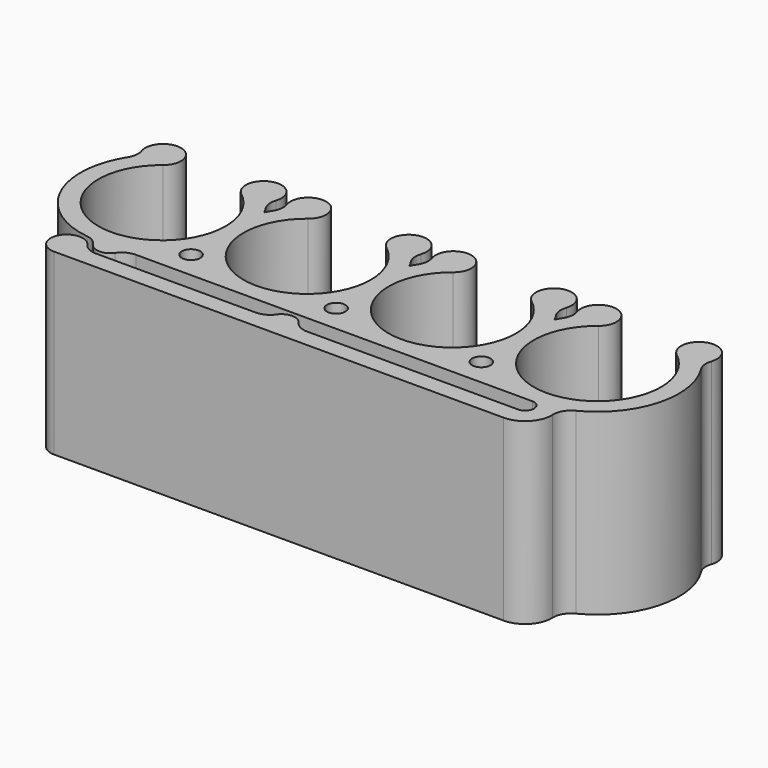
from build123d import *

# Parameters (mm, degrees)
F1_R     = 1.03125
F2_DEPTH = 10
F3_R     = 2


with BuildPart() as f2:
    # F1 (on Top) → F2 (new body, symmetric)
    with BuildSketch(Plane.XY):
        with BuildLine():
            ThreePointArc((-19.9828767123, 14.7352475904), (-17.9695529655, 12.2452360949), (-17.25, 9.125))
            ThreePointArc((-17.25, 9.125), (-27.4952360949, 2.7195529655), (-28.7671232877, 14.7352475904))
            ThreePointArc((-28.7671232877, 14.7352475904), (-29.8675330526, 18.3056622368), (-31.4302114786, 14.9120213402))
            ThreePointArc((-31.4302114786, 14.9120213402), (-32.6233996851, 5.2224972601), (-24.375, 0))
            Line((-24.375, 0), (-21.375, 0))
            Line((-21.375, 0), (24.375, 0))
            ThreePointArc((24.375, 0), (25.7175606637, 0.099305796), (27.0308996167, 0.3950617284))
            ThreePointArc((27.0308996167, 0.3950617284), (33.107808756, 6.4785540378), (31.4302114786, 14.9120213402))
            ThreePointArc((31.4302114786, 14.9120213402), (29.8675330526, 18.3056622368), (28.7671232877, 14.7352475904))
            ThreePointArc((28.7671232877, 14.7352475904), (30.7804470345, 12.2452360949), (31.5, 9.125))
            ThreePointArc((31.5, 9.125), (21.2547639051, 2.7195529655), (19.9828767123, 14.7352475904))
            ThreePointArc((19.9828767123, 14.7352475904), (18.8824669474, 18.3056622368), (17.3197885214, 14.9120213402))
            ThreePointArc((17.3197885214, 14.9120213402), (16.7410654482, 14.1238666974), (16.25, 13.2783119315))
            ThreePointArc((16.25, 13.2783119315), (15.7589345518, 14.1238666974), (15.1802114786, 14.9120213402))
            ThreePointArc((15.1802114786, 14.9120213402), (13.6175330526, 18.3056622368), (12.5171232877, 14.7352475904))
            ThreePointArc((12.5171232877, 14.7352475904), (14.5304470345, 12.2452360949), (15.25, 9.125))
            ThreePointArc((15.25, 9.125), (5.0047639051, 2.7195529655), (3.7328767123, 14.7352475904))
            ThreePointArc((3.7328767123, 14.7352475904), (2.6324669474, 18.3056622368), (1.0697885214, 14.9120213402))
            ThreePointArc((1.0697885214, 14.9120213402), (0.4910654482, 14.1238666974), (0, 13.2783119315))
            ThreePointArc((0, 13.2783119315), (-0.4910654482, 14.1238666974), (-1.0697885214, 14.9120213402))
            ThreePointArc((-1.0697885214, 14.9120213402), (-2.6324669474, 18.3056622368), (-3.7328767123, 14.7352475904))
            ThreePointArc((-3.7328767123, 14.7352475904), (-1.7195529655, 12.2452360949), (-1, 9.125))
            ThreePointArc((-1, 9.125), (-11.2452360949, 2.7195529655), (-12.5171232877, 14.7352475904))
            ThreePointArc((-12.5171232877, 14.7352475904), (-13.6175330526, 18.3056622368), (-15.1802114786, 14.9120213402))
            ThreePointArc((-15.1802114786, 14.9120213402), (-15.7589345518, 14.1238666974), (-16.25, 13.2783119315))
            ThreePointArc((-16.25, 13.2783119315), (-16.7410654482, 14.1238666974), (-17.3197885214, 14.9120213402))
            ThreePointArc((-17.3197885214, 14.9120213402), (-18.8824669474, 18.3056622368), (-19.9828767123, 14.7352475904))
        make_face()
        with Locations((-16.25, 3.03125)):
            Circle(F1_R, mode=Mode.SUBTRACT)
        with Locations((0, 3.03125)):
            Circle(F1_R, mode=Mode.SUBTRACT)
        with Locations((16.25, 3.03125)):
            Circle(F1_R, mode=Mode.SUBTRACT)
        with BuildLine():
            ThreePointArc((27.0308996167, 0.3950617284), (25.7175606637, 0.099305796), (24.375, 0))
            ThreePointArc((24.375, 0), (25.375, -1), (24.375, -2))
            Line((24.375, -2), (-0.6061253537, -2))
            Line((-0.6061253537, -2), (-3.6061253537, -2))
            Line((-3.6061253537, -2), (-24.1903478035, -2))
            ThreePointArc((-24.1903478035, -2), (-27.3314384085, -0.985167759), (-25.9871463178, -4))
            Line((-25.9871463178, -4), (24.375, -4))
            ThreePointArc((24.375, -4), (26.9426044463, -2.5515822271), (27.0308996167, 0.3950617284))
        make_face()
        with BuildLine():
            Line((-21.375, 0), (-24.375, 0))
            ThreePointArc((-24.375, 0), (-22.875, -1.5), (-21.375, 0))
        make_face()
        with BuildLine():
            Line((-3.6061253537, -2), (-0.6061253537, -2))
            ThreePointArc((-0.6061253537, -2), (-2.1061253537, -0.5), (-3.6061253537, -2))
        make_face()
    extrude(amount=F2_DEPTH, both=True)

    # F3
    f3_edges = [f2.edges().sort_by_distance(p)[0] for p in [
        (31.430211, 14.912021, 0),
        (15.180211, 14.912021, 0),
        (17.319789, 14.912021, 0),
        (1.069789, 14.912021, 0),
        (-15.180211, 14.912021, 0),
        (-31.430211, 14.912021, 0),
        (-17.319789, 14.912021, 0),
        (-1.069789, 14.912021, 0),
        (-24.375, 0, 0),
        (27.0309, 0.395062, 0),
        (-24.190348, -2, 0),
        (-0.606125, -2, 0),
        (-3.606125, -2, 0),
        (-21.375, 0, 0),
    ]]
    fillet(f3_edges, radius=F3_R)


solid = f2.part
